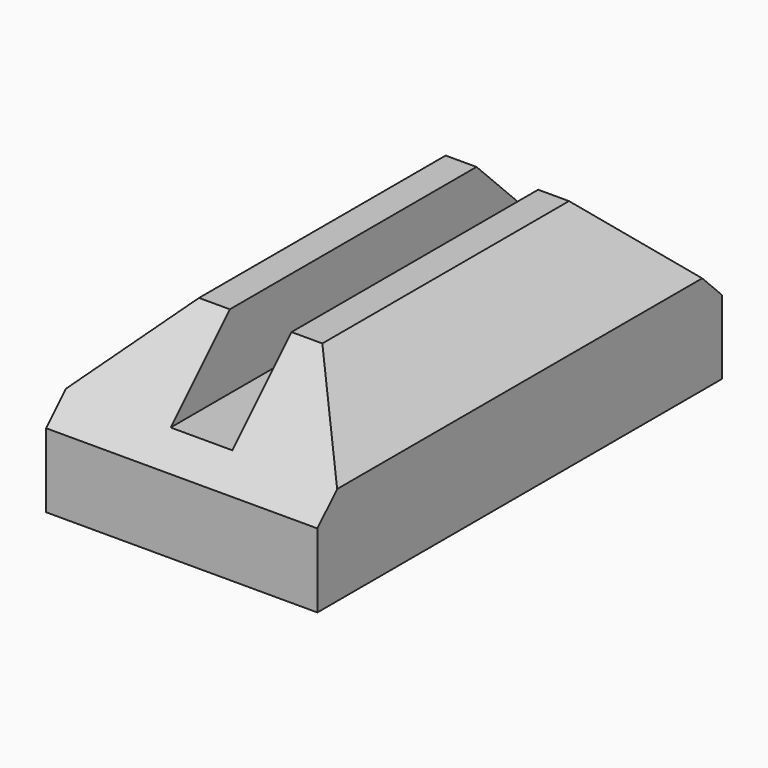
from build123d import *

# Parameters (mm, degrees)
F1_DEPTH   = 130.175
F2_C1_SIZE = 25.4
F2_C2_SIZE = 25.4


with BuildPart() as f1:
    # F0 (on Front) → F1 (new body)
    with BuildSketch(Plane.XZ):
        Polygon((0, 25.4), (0, 0), (69.85, 0), (69.85, 25.4), (50.8, 44.45), (42.8625, 44.45), (42.8625, 25.4), (26.9875, 25.4), (26.9875, 44.45), (19.05, 44.45), align=None)
    extrude(amount=F1_DEPTH)

    # F2: chamfer of 25.4 on 4 edges, made by hand

    # F2_c1
    f2_c1_edges = [f1.edges().sort_by_distance(p)[0] for p in [
        (46.83125, 0, 44.45),
    ]]
    chamfer(f2_c1_edges, length=F2_C1_SIZE)

    # F2_c2
    f2_c2_edges = [f1.edges().sort_by_distance(p)[0] for p in [
        (46.83125, -130.175, 44.45),
    ]]
    chamfer(f2_c2_edges, length=F2_C2_SIZE)


solid = f1.part
